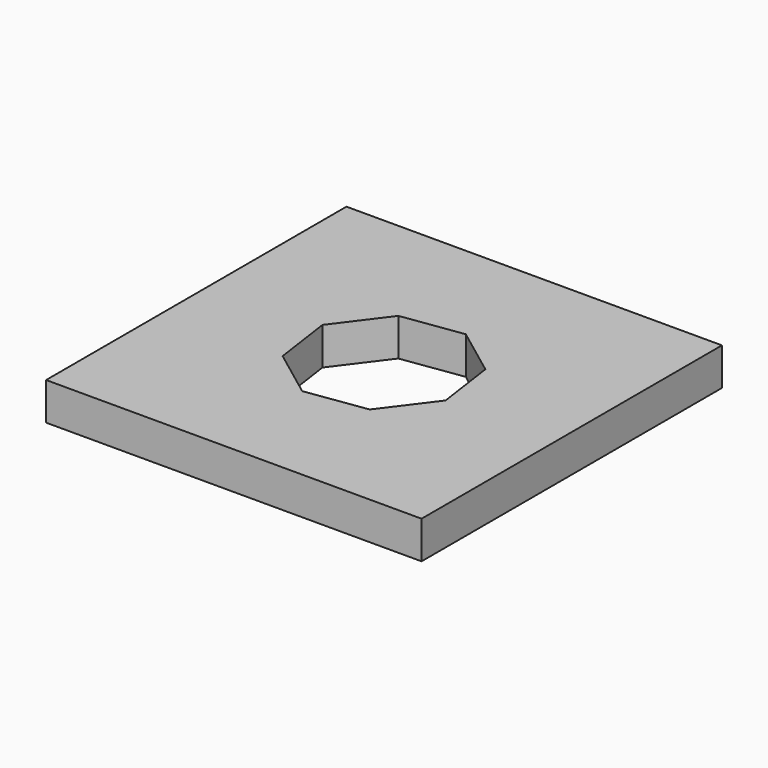
from build123d import *

# Parameters (mm, degrees)
F0_W     = 100
F0_H     = 100
F1_DEPTH = 10
F3_DEPTH = 39.624


# Not quite as in the source:
# - a feature names something its author has since deleted; it is built from what else it names


with BuildPart() as f1:
    # F0 (on Top) → F1 (new body)
    with BuildSketch(Plane.XY):
        Rectangle(F0_W, F0_H)
    extrude(amount=-F1_DEPTH)

    # F2 (on face) → F3 (cut)
    with BuildSketch(Plane.XY):
        Polygon((10.8499823283, -18.3243404083), (20.6293614436, -5.2851692833), (18.3243404083, 10.8499823283), (5.2851692833, 20.6293614436), (-10.8499823283, 18.3243404083), (-20.6293614436, 5.2851692833), (-18.3243404083, -10.8499823283), (-5.2851692833, -20.6293614436), align=None)
    extrude(amount=-F3_DEPTH, mode=Mode.SUBTRACT)


solid = f1.part
